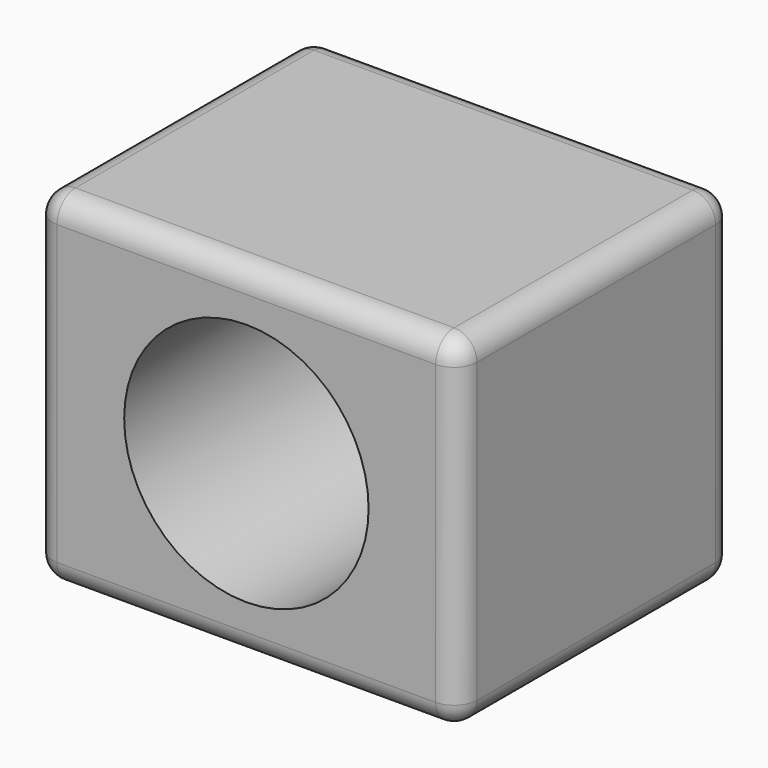
from build123d import *

# Parameters (mm, degrees)
F0_W         = 94.0244570374
F0_H         = 76.03880018
F1_DEPTH     = 76.2
F2_R         = 27.0679011962
F3_DEPTH     = 101.6
F4_R         = 5.08
F5_T1_DEPTH  = 83.8644570374
F5_T3_DEPTH  = 65.87880018
F5_T5_DEPTH  = 66.04
F5_S9_W      = 5.08
F5_S9_H      = 5.08
F5_T10_DEPTH = 5.08
F5_S15_W     = 5.08
F5_S15_H     = 5.08
F5_T16_DEPTH = 5.08
F5_S21_W     = 5.08
F5_S21_H     = 5.08
F5_T22_DEPTH = 5.08
F5_S27_W     = 5.08
F5_S27_H     = 5.08
F5_T28_DEPTH = 5.08


# Not quite as in the source:
# - a fillet or chamfer that OpenCascade refuses, or shapes differently, is made with other operations: its cross-section is extruded or revolved along the edge and cut away or added


with BuildPart() as f1:
    # F0 (on Front) → F1 (new body)
    with BuildSketch(Plane.XZ):
        Rectangle(F0_W, F0_H)
    extrude(amount=F1_DEPTH)

    # F2 (on face) → F3 (cut)
    with BuildSketch(Plane(origin=(0, 0, 0), x_dir=(-1, 0, 0), z_dir=(0, 1, 0))):
        Circle(F2_R)
    extrude(amount=-F3_DEPTH, mode=Mode.SUBTRACT)

    # F4
    f4_edges = [f1.edges().sort_by_distance(p)[0] for p in [
        (0, -76.2, 38.0194),
        (47.012229, -38.1, 38.0194),
        (0, 0, 38.0194),
        (-47.012229, -38.1, 38.0194),
        (47.012229, -76.2, 0),
        (47.012229, 0, 0),
        (47.012229, -38.1, -38.0194),
        (0, -76.2, -38.0194),
        (-47.012229, -76.2, 0),
    ]]
    fillet(f4_edges, radius=F4_R)

    # F5: fillet of radius 5.08 on 3 edges, made by hand

    # F5_s2 → F5_t1 (cut)
    with BuildSketch(Plane.YZ.offset(-41.9322285187)):
        with BuildLine():
            ThreePointArc((0, -32.93940009), (-1.4878975516, -36.5315025384), (-5.08, -38.01940009))
            Line((-5.08, -38.01940009), (0, -38.01940009))
            Line((0, -38.01940009), (0, -32.93940009))
        make_face()
    extrude(amount=F5_T1_DEPTH, mode=Mode.SUBTRACT)

    # F5_s4 → F5_t3 (cut)
    with BuildSketch(Plane.XY.offset(-32.93940009)):
        with BuildLine():
            ThreePointArc((-41.9322285187, 0), (-45.5243309672, -1.4878975516), (-47.0122285187, -5.08))
            Line((-47.0122285187, -5.08), (-47.0122285187, 0))
            Line((-47.0122285187, 0), (-41.9322285187, 0))
        make_face()
    extrude(amount=F5_T3_DEPTH, mode=Mode.SUBTRACT)

    # F5_s6 → F5_t5 (cut)
    with BuildSketch(Plane.XZ.offset(5.08)):
        with BuildLine():
            ThreePointArc((-41.9322285187, -38.01940009), (-45.5243309672, -36.5315025384), (-47.0122285187, -32.93940009))
            Line((-47.0122285187, -32.93940009), (-47.0122285187, -38.01940009))
            Line((-47.0122285187, -38.01940009), (-41.9322285187, -38.01940009))
        make_face()
    extrude(amount=F5_T5_DEPTH, mode=Mode.SUBTRACT)


with BuildPart() as f5_tool8:
    # F5_s9 → F5_t10 (new body)
    with BuildSketch(Plane.XY.offset(-32.93940009)):
        with Locations((-44.4722285187, -73.66)):
            Rectangle(F5_S9_W, F5_S9_H)
    extrude(amount=-F5_T10_DEPTH)

    # F5_s11 → F5_t12 (revolve, cut)
    with BuildSketch(Plane(origin=(-41.9322285187, -71.12, -32.93940009), x_dir=(0.7071067812, 0.7071067812, 0), z_dir=(-0.7071067812, 0.7071067812, 0))):
        with BuildLine():
            ThreePointArc((0, -5.08), (5.08, 0), (0, 5.08))
            Line((0, 5.08), (0, -5.08))
        make_face()
    revolve(axis=Axis((-41.9322285187, -71.12, -32.93940009), (0, 0, -1)), mode=Mode.SUBTRACT)


with BuildPart() as f1_1:
    add(f1.part)

    # F5_t7: cut F5_tool8
    add(f5_tool8.part, mode=Mode.SUBTRACT)


with BuildPart() as f5_tool14:
    # F5_s15 → F5_t16 (new body)
    with BuildSketch(Plane.XZ.offset(5.08)):
        with Locations((-44.4722285187, 35.47940009)):
            Rectangle(F5_S15_W, F5_S15_H)
    extrude(amount=-F5_T16_DEPTH)

    # F5_s17 → F5_t18 (revolve, cut)
    with BuildSketch(Plane(origin=(-41.9322285187, -5.08, 32.93940009), x_dir=(0.7071067812, 0, -0.7071067812), z_dir=(0.7071067812, 0, 0.7071067812))):
        with BuildLine():
            ThreePointArc((0, -5.08), (5.08, 0), (0, 5.08))
            Line((0, 5.08), (0, -5.08))
        make_face()
    revolve(axis=Axis((-41.9322285187, -5.08, 32.93940009), (0, 1, 0)), mode=Mode.SUBTRACT)


with BuildPart() as f1_2:
    add(f1_1.part)

    # F5_t13: cut F5_tool14
    add(f5_tool14.part, mode=Mode.SUBTRACT)


with BuildPart() as f5_tool20:
    # F5_s21 → F5_t22 (new body)
    with BuildSketch(Plane.XZ.offset(5.08)):
        with Locations((44.4722285187, -35.47940009)):
            Rectangle(F5_S21_W, F5_S21_H)
    extrude(amount=-F5_T22_DEPTH)

    # F5_s23 → F5_t24 (revolve, cut)
    with BuildSketch(Plane(origin=(41.9322285187, -5.08, -32.93940009), x_dir=(-0.7071067812, 0, 0.7071067812), z_dir=(-0.7071067812, 0, -0.7071067812))):
        with BuildLine():
            ThreePointArc((0, -5.08), (5.08, 0), (0, 5.08))
            Line((0, 5.08), (0, -5.08))
        make_face()
    revolve(axis=Axis((41.9322285187, -5.08, -32.93940009), (0, 1, 0)), mode=Mode.SUBTRACT)


with BuildPart() as f1_3:
    add(f1_2.part)

    # F5_t19: cut F5_tool20
    add(f5_tool20.part, mode=Mode.SUBTRACT)


with BuildPart() as f5_tool26:
    # F5_s27 → F5_t28 (new body)
    with BuildSketch(Plane.XZ.offset(5.08)):
        with Locations((-44.4722285187, -35.47940009)):
            Rectangle(F5_S27_W, F5_S27_H)
    extrude(amount=-F5_T28_DEPTH)

    # F5_s29 → F5_t30 (revolve, cut)
    with BuildSketch(Plane(origin=(-41.9322285187, -5.08, -32.93940009), x_dir=(0.7071067812, 0, 0.7071067812), z_dir=(-0.7071067812, 0, 0.7071067812))):
        with BuildLine():
            ThreePointArc((0, -5.08), (5.08, 0), (0, 5.08))
            Line((0, 5.08), (0, -5.08))
        make_face()
    revolve(axis=Axis((-41.9322285187, -5.08, -32.93940009), (0, 1, 0)), mode=Mode.SUBTRACT)


with BuildPart() as f1_4:
    add(f1_3.part)

    # F5_t25: cut F5_tool26
    add(f5_tool26.part, mode=Mode.SUBTRACT)


solid = f1_4.part
